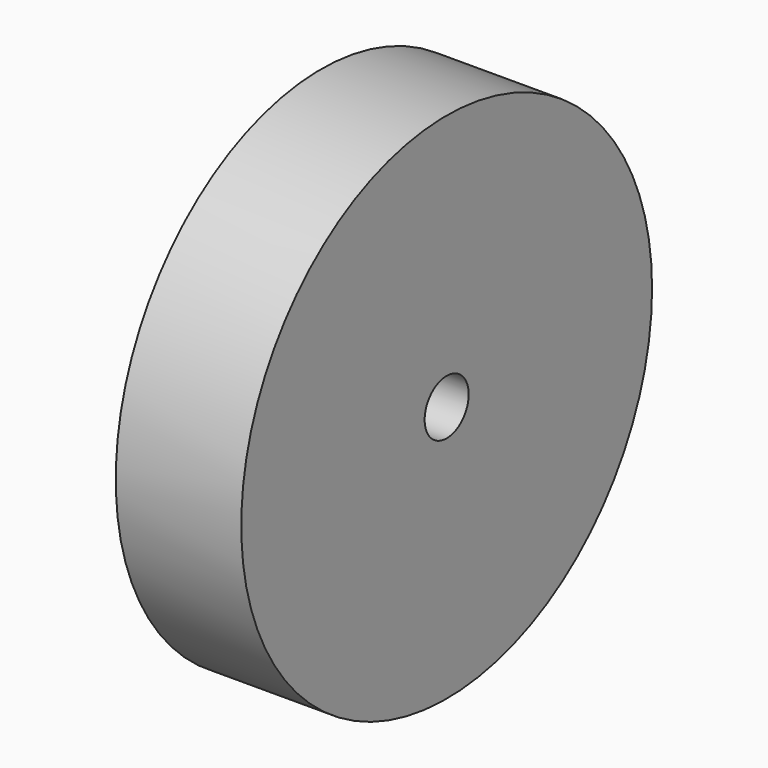
from build123d import *

# Parameters (mm, degrees)
F0_R          = 103.9250934244
F0_R_2        = 11.1470485127
F1_DEPTH      = 25.4
F1_DEPTH_BACK = 25.4


# Not quite as in the source:
# - the program builds the solid bodies; features that only make, move or delete a surface that nothing else refers to are left out


with BuildPart() as f1:
    # F0 (on Right) → F1 (new body, two sides)
    with BuildSketch(Plane.YZ) as f1_sk:
        Circle(F0_R)
        Circle(F0_R_2, mode=Mode.SUBTRACT)
    extrude(amount=F1_DEPTH)
    extrude(f1_sk.sketch, amount=-F1_DEPTH_BACK)


solid = f1.part
